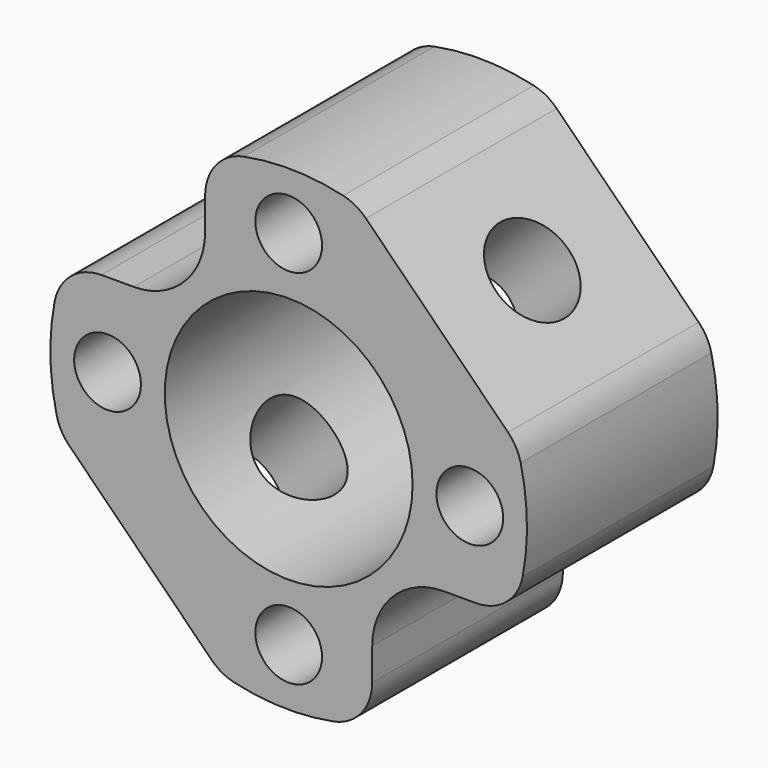
from build123d import *

# Parameters (mm, degrees)
F0_R     = 25
F0_R_2   = 3.5
F1_DEPTH = 25
F3_DEPTH = 25.001
F4_R     = 5
F5_R     = 13
F6_DEPTH = 25.001
F7_R     = 4.75
F8_DEPTH = 57.3563390593


with BuildPart() as f1:
    # F0 (on Front) → F1 (new body)
    with BuildSketch(Plane.XZ):
        Circle(F0_R)
        with Locations((0, -19)):
            Circle(F0_R_2, mode=Mode.SUBTRACT)
        with Locations((-19, 0)):
            Circle(F0_R_2, mode=Mode.SUBTRACT)
        with Locations((19, 0)):
            Circle(F0_R_2, mode=Mode.SUBTRACT)
        with Locations((0, 19)):
            Circle(F0_R_2, mode=Mode.SUBTRACT)
    extrude(amount=F1_DEPTH)

    # F2 (on Front) → F3 (cut, through all)
    with BuildSketch(Plane.XZ):
        with BuildLine():
            Line((-23.7634559673, 8.7634559673), (-16.2634559673, 8.7634559673))
            ThreePointArc((-16.2634559673, 8.7634559673), (-10.9601551084, 10.9601551084), (-8.7634559673, 16.2634559673))
            Line((-8.7634559673, 16.2634559673), (-8.7634559673, 23.7634559673))
            Line((-8.7634559673, 23.7634559673), (-23.7634559673, 23.7634559673))
            Line((-23.7634559673, 23.7634559673), (-23.7634559673, 8.7634559673))
        make_face()
        Polygon((1.4142135624, 29.6984848098), (29.6984848098, 1.4142135624), (61.3951798296, 33.6381491506), (33.3745288664, 61.6588001138), align=None)
        Polygon((-1.4142135624, -29.6984848098), (-29.6984848098, -1.4142135624), (-61.6588001138, -33.3745288664), (-33.6381491506, -61.3951798296), align=None)
        with BuildLine():
            ThreePointArc((16.2634559673, -8.7634559673), (10.9601551084, -10.9601551084), (8.7634559673, -16.2634559673))
            Line((8.7634559673, -16.2634559673), (8.7634559673, -23.7634559673))
            Line((8.7634559673, -23.7634559673), (23.7634559673, -23.7634559673))
            Line((23.7634559673, -23.7634559673), (23.7634559673, -8.7634559673))
            Line((23.7634559673, -8.7634559673), (16.2634559673, -8.7634559673))
        make_face()
    extrude(amount=F3_DEPTH, mode=Mode.SUBTRACT)

    # F4
    f4_edges = [f1.edges().sort_by_distance(p)[0] for p in [
        (-8.763456, -12.5, 23.413711),
        (-23.413711, -12.5, 8.763456),
        (8.763456, -12.5, -23.413711),
        (23.413711, -12.5, -8.763456),
        (23.952777, -12.5, 7.159921),
        (7.159921, -12.5, 23.952777),
        (-23.952777, -12.5, -7.159921),
        (-7.159921, -12.5, -23.952777),
    ]]
    fillet(f4_edges, radius=F4_R)

    # F5 (on Front) → F6 (cut, through all)
    with BuildSketch(Plane.XZ):
        Circle(F5_R)
    extrude(amount=F6_DEPTH, mode=Mode.SUBTRACT)

    # F7 (on face) → F8 (cut, through all)
    with BuildSketch(Plane(origin=(15.5563491861, 0, 15.5563491861), x_dir=(0.7071067812, 0, -0.7071067812), z_dir=(0.7071067812, 0, 0.7071067812))):
        with Locations((0, -12.5)):
            Circle(F7_R)
    extrude(amount=-F8_DEPTH, mode=Mode.SUBTRACT)


solid = f1.part
